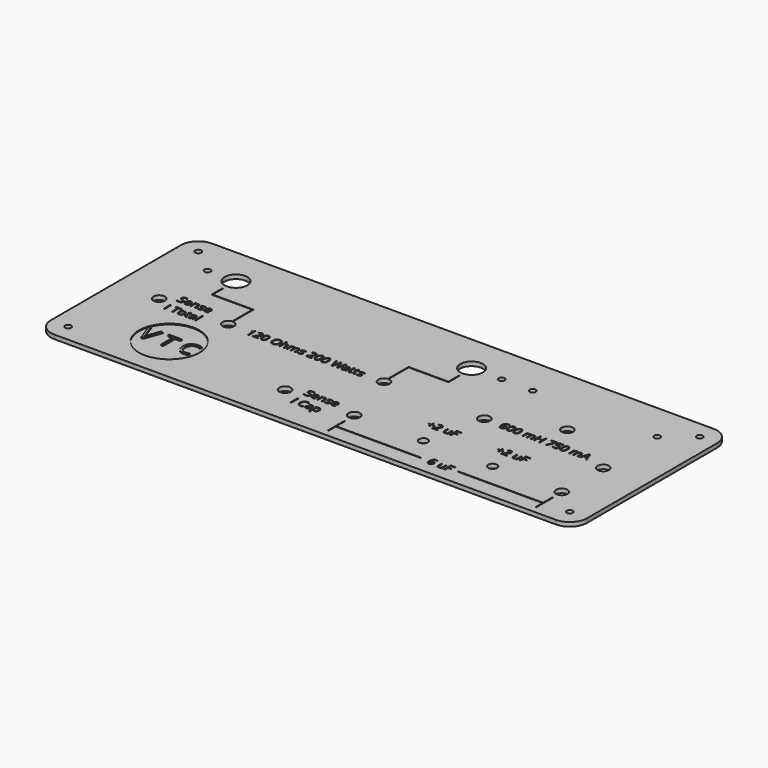
from build123d import *

# Parameters (mm, degrees)
F1_DEPTH     = 2.9972
F2_D         = 4.4958
F3_D         = 16.66748
F4_D         = 8.4328
F5_D         = 6.5278
F6_W         = 62.3732725377
F6_H         = 0.508
F6_W_2       = 62.23
F6_R         = 22.225
F6_W_3       = 0.508
F6_H_2       = 17.78
F6_TEXT_SIZE = 8.8194444444
F7_DEPTH     = 0.635


# Not quite as in the source:
# - Text() gives the source's letters only with a copy of the font that has no kerning and outlines rounded to 1/6400 em; it was checked with that copy


with BuildPart() as f1:
    # F0 (on Top) → F1 (new body)
    with BuildSketch(Plane.XY):
        with BuildLine():
            ThreePointArc((196.85, 59.69), (193.1302561211, 68.6702561211), (184.15, 72.39))
            Line((184.15, 72.39), (-184.15, 72.39))
            ThreePointArc((-184.15, 72.39), (-193.1302561211, 68.6702561211), (-196.85, 59.69))
            Line((-196.85, 59.69), (-196.85, -59.69))
            ThreePointArc((-196.85, -59.69), (-193.1302561211, -68.6702561211), (-184.15, -72.39))
            Line((-184.15, -72.39), (184.15, -72.39))
            ThreePointArc((184.15, -72.39), (193.1302561211, -68.6702561211), (196.85, -59.69))
            Line((196.85, -59.69), (196.85, 59.69))
        make_face()
    extrude(amount=F1_DEPTH)

    # F2 (through all)
    with Locations(Plane(origin=(0, 0, 0), x_dir=(1, 0, 0), z_dir=(0, 0, -1))):
        with Locations((165.1, -44.45), (73.66, -44.45), (50.8, -44.45), (-165.1, -44.45), (-184.15, -59.69), (-184.15, 59.69), (184.15, 59.69), (184.15, -59.69)):
            Hole(F2_D / 2)

    # F3 (through all)
    with Locations(Plane(origin=(0, 0, 0), x_dir=(1, 0, 0), z_dir=(0, 0, -1))):
        with Locations((28.7782, -44.45), (-144.272, -44.45)):
            Hole(F3_D / 2)

    # F4 (through all)
    with Locations(Plane(origin=(0, 0, 0), x_dir=(1, 0, 0), z_dir=(0, 0, -1))):
        with Locations((165.1, 5.08), (73.66, 0), (0, 0), (-114.3, 0), (165.1, 43.18), (-38.1, 43.18), (-165.1, 0), (119.38, -19.05), (12.7, 43.18)):
            Hole(F4_D / 2)

    # F5 (through all)
    with Locations(Plane(origin=(0, 0, 0), x_dir=(1, 0, 0), z_dir=(0, 0, -1))):
        with Locations((63.5, 43.18), (114.3, 43.18)):
            Hole(F5_D / 2)

    # F6 (on face) → F7 (cut)
    with BuildSketch(Plane.XY.offset(2.9972)):
        with Locations((44.3946362689, -60.5896986804)):
            Rectangle(F6_W, F6_H)
        Polygon((13.208, -60.8436986804), (13.208, -60.3356986804), (13.208, -52.07), (12.7, -52.07), (12.7, -67.31), (13.208, -67.31), align=None)
        Polygon((165.608, -52.07), (165.1, -52.07), (165.1, -60.3356986804), (165.1, -60.8436986804), (165.1, -67.31), (165.608, -67.31), align=None)
        with Locations((133.985, -60.5896986804)):
            Rectangle(F6_W_2, F6_H)
        with Locations((-127.3822188377, -37.9314981401)):
            Circle(F6_R)
        with BuildLine():
            Line((-141.7332698486, -39.3650812587), (-138.8929860087, -31.3720219469))
            Line((-138.8929860087, -31.3720219469), (-137.3395357476, -31.3720219469))
            Line((-137.3395357476, -31.3720219469), (-141.8176077787, -43.8023446139))
            Line((-141.8176077787, -43.8023446139), (-143.2459114338, -43.8023446139))
            Line((-143.2459114338, -43.8023446139), (-147.7022188377, -31.3720219469))
            Line((-147.7022188377, -31.3720219469), (-146.1705332038, -31.3720219469))
            Line((-146.1705332038, -31.3720219469), (-143.3139258936, -39.4140516698))
            add(Edge.make_bspline(
                [(-143.3139258936, -39.4140516698), (-142.8215012049, -40.801546649), (-142.5331198954, -42.1101448549)],
                knots=[0, 0, 0, 1, 1, 1], degree=2))
            add(Edge.make_bspline(
                [(-142.5331198954, -42.1101448549), (-142.2256945373, -40.7335321893), (-141.7332698486, -39.3650812587)],
                knots=[0, 0, 0, 1, 1, 1], degree=2))
        make_face(mode=Mode.SUBTRACT)
        Polygon((-127.2815574373, -32.6561349473), (-127.2815574373, -43.8023446139), (-128.7261845627, -43.8023446139), (-128.7261845627, -32.6561349473), (-132.6628614941, -32.6561349473), (-132.6628614941, -31.3720219469), (-123.344880506, -31.3720219469), (-123.344880506, -32.6561349473), align=None, mode=Mode.SUBTRACT)
        with BuildLine():
            add(Edge.make_bspline(
                [(-108.8033890078, -33.148559636), (-110.2153691925, -32.4874590871), (-111.6273493773, -32.4874590871)],
                knots=[0, 0, 0, 1, 1, 1], degree=2))
            add(Edge.make_bspline(
                [(-111.6273493773, -32.4874590871), (-113.6759449055, -32.4874590871), (-114.8621170838, -33.85182915)],
                knots=[0, 0, 0, 1, 1, 1], degree=2))
            add(Edge.make_bspline(
                [(-114.8621170838, -33.85182915), (-116.0482892622, -35.2161992129), (-116.0482892622, -37.5885435696)],
                knots=[0, 0, 0, 1, 1, 1], degree=2))
            add(Edge.make_bspline(
                [(-116.0482892622, -37.5885435696), (-116.0482892622, -40.0261818077), (-114.9042860489, -41.3579049299)],
                knots=[0, 0, 0, 1, 1, 1], degree=2))
            add(Edge.make_bspline(
                [(-114.9042860489, -41.3579049299), (-113.7602828356, -42.6896280522), (-111.6436728476, -42.6896280522)],
                knots=[0, 0, 0, 1, 1, 1], degree=2))
            add(Edge.make_bspline(
                [(-111.6436728476, -42.6896280522), (-110.3432363769, -42.6896280522), (-108.6755218234, -42.221688569)],
                knots=[0, 0, 0, 1, 1, 1], degree=2))
            Line((-108.6755218234, -42.221688569), (-108.6755218234, -43.4867575206))
            add(Edge.make_bspline(
                [(-108.6755218234, -43.4867575206), (-109.967796559, -43.9737410526), (-111.8640396973, -43.9737410526)],
                knots=[0, 0, 0, 1, 1, 1], degree=2))
            add(Edge.make_bspline(
                [(-111.8640396973, -43.9737410526), (-114.6091032935, -43.9737410526), (-116.1013405408, -42.3060264991)],
                knots=[0, 0, 0, 1, 1, 1], degree=2))
            add(Edge.make_bspline(
                [(-116.1013405408, -42.3060264991), (-117.5935777881, -40.6383119456), (-117.5935777881, -37.5694995209)],
                knots=[0, 0, 0, 1, 1, 1], degree=2))
            add(Edge.make_bspline(
                [(-117.5935777881, -37.5694995209), (-117.5935777881, -35.6487711771), (-116.8753450929, -34.2041440516)],
                knots=[0, 0, 0, 1, 1, 1], degree=2))
            add(Edge.make_bspline(
                [(-116.8753450929, -34.2041440516), (-116.1571123978, -32.7595169262), (-114.80090407, -31.9773506388)],
                knots=[0, 0, 0, 1, 1, 1], degree=2))
            add(Edge.make_bspline(
                [(-114.80090407, -31.9773506388), (-113.4446957423, -31.1951843515), (-111.6083053286, -31.1951843515)],
                knots=[0, 0, 0, 1, 1, 1], degree=2))
            add(Edge.make_bspline(
                [(-111.6083053286, -31.1951843515), (-109.6549300441, -31.1951843515), (-108.1912588699, -31.9079758899)],
                knots=[0, 0, 0, 1, 1, 1], degree=2))
            Line((-108.1912588699, -31.9079758899), (-108.8033890078, -33.148559636))
        make_face(mode=Mode.SUBTRACT)
        Polygon((-144.272, 23.13891481), (-144.272, 22.63091481), (-114.808, 22.63091481), (-114.3, 22.63091481), (-114.3, 23.13891481), align=None)
        Polygon((-144.78, 22.63091481), (-144.272, 22.63091481), (-144.272, 23.13891481), (-144.272, 32.79091481), (-144.78, 32.79091481), align=None)
        with Locations((-114.554, 13.74091481)):
            Rectangle(F6_W_3, F6_H_2)
        Polygon((-0.508, 23.13891481), (-0.508, 22.63091481), (0, 22.63091481), (28.7782, 22.63091481), (28.7782, 23.13891481), align=None)
        with Locations((-0.254, 13.74091481)):
            Rectangle(F6_W_3, F6_H_2)
        Polygon((28.7782, 23.13891481), (28.7782, 22.63091481), (29.2862, 22.63091481), (29.2862, 32.79091481), (28.7782, 32.79091481), align=None)
        with Locations((-99.7047621019, -3.1467200024)):
            Text('120 Ohms 200 Watts', F6_TEXT_SIZE, font='Open Sans', text_align=(TextAlign.LEFT, TextAlign.BOTTOM))
        with Locations((85.7776195201, -3.1467200024)):
            Text('600 mH 750 mA', F6_TEXT_SIZE, font='Open Sans', text_align=(TextAlign.LEFT, TextAlign.BOTTOM))
        with Locations((-156.1655379076, 3.9045855174)):
            Text('Sense', F6_TEXT_SIZE, font='Open Sans', text_align=(TextAlign.LEFT, TextAlign.BOTTOM))
        with Locations((-156.1655379076, -8.089858927)):
            Text('I Total', F6_TEXT_SIZE, font='Open Sans', text_align=(TextAlign.LEFT, TextAlign.BOTTOM))
        with Locations((-26.7422658932, -41.4231153899)):
            Text('Sense', F6_TEXT_SIZE, font='Open Sans', text_align=(TextAlign.LEFT, TextAlign.BOTTOM))
        with Locations((-26.7422658932, -53.4175598344)):
            Text('I Cap', F6_TEXT_SIZE, font='Open Sans', text_align=(TextAlign.LEFT, TextAlign.BOTTOM))
        with Locations((102.9318739149, -27.94)):
            Text('+2 uF', F6_TEXT_SIZE, font='Open Sans', text_align=(TextAlign.LEFT, TextAlign.BOTTOM))
        with Locations((81.2633287177, -63.5106986804)):
            Text('6 uF', F6_TEXT_SIZE, font='Open Sans', text_align=(TextAlign.LEFT, TextAlign.BOTTOM))
        with Locations((52.1318739149, -27.94)):
            Text('+2 uF', F6_TEXT_SIZE, font='Open Sans', text_align=(TextAlign.LEFT, TextAlign.BOTTOM))
    extrude(amount=-F7_DEPTH, mode=Mode.SUBTRACT)


solid = f1.part
